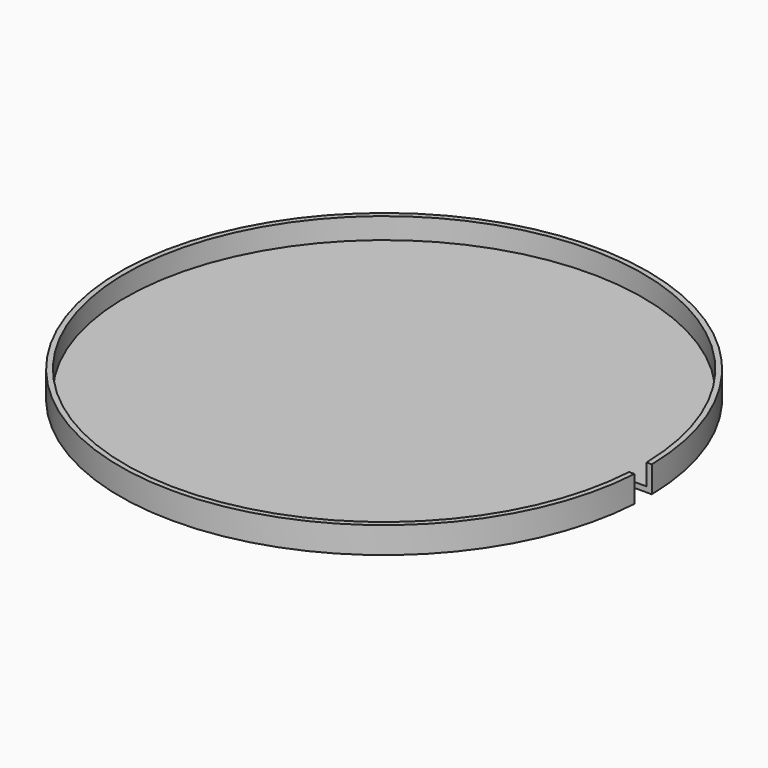
from build123d import *

# Parameters (mm, degrees)
F0_R     = 50
F1_DEPTH = 5
F2_T     = -1
F3_W     = 4
F3_H     = 4
F4_DEPTH = 6


# Not quite as in the source:
# - the program builds the solid bodies; features that only make, move or delete a surface that nothing else refers to are left out


with BuildPart() as f1:
    # F0 (on Top) → F1 (new body)
    with BuildSketch(Plane.XY):
        Circle(F0_R)
    extrude(amount=F1_DEPTH)

    # F2
    f2_openings = [f1.faces().sort_by_distance(p)[0] for p in [
        (0, 0, 5),
    ]]
    offset(amount=F2_T, openings=f2_openings)

    # F3 (on Top) → F4 (cut)
    with BuildSketch(Plane.XY):
        with Locations((48.6989099085, -1.1040147878)):
            Rectangle(F3_W, F3_H)
    extrude(amount=F4_DEPTH, mode=Mode.SUBTRACT)


solid = f1.part
